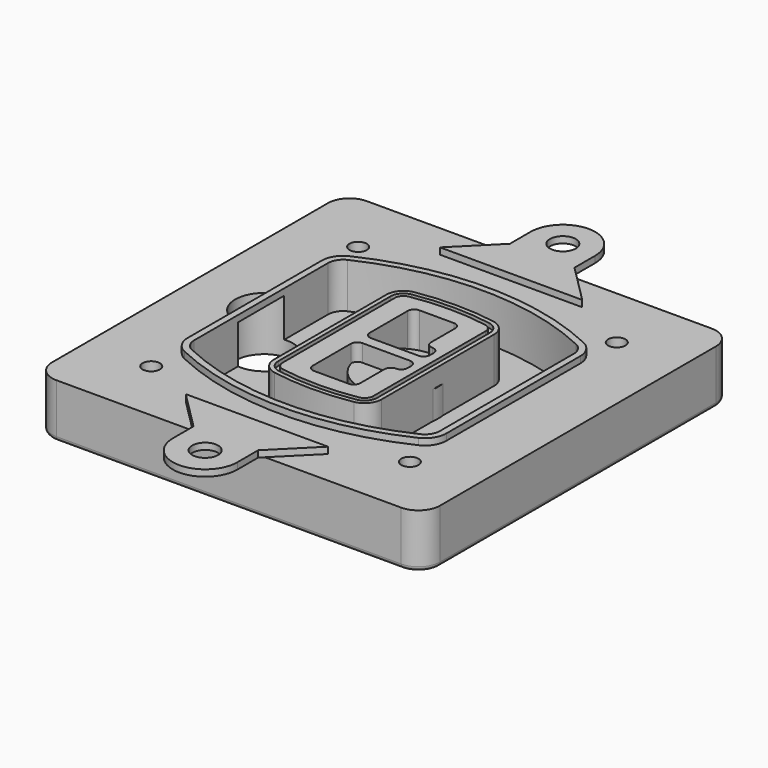
from build123d import *

# Parameters (mm, degrees)
F0_R      = 4
F1_DEPTH  = 25
F2_DEPTH  = 3
F3_DEPTH  = 18
F5_DEPTH  = 21
F6_DEPTH  = 2
F8_DEPTH  = 20
F9_DEPTH  = 16
F10_DEPTH = 25
F7_R      = 6
F7_R_2    = 4
F11_DEPTH = 6
F13_DEPTH = 9
F15_R     = 2
F16_R     = 6
F17_DEPTH = 3


# Not quite as in the source:
# - a feature of the source that left no trace in its solid (it failed there, or was rolled back) is left out
# - a feature names something its author has since deleted; it is built from what else it names


with BuildPart() as f1:
    # F0 (on Top) → F1 (new body)
    with BuildSketch(Plane.XY):
        with BuildLine():
            ThreePointArc((-90, -80), (-87.0710678119, -87.0710678119), (-80, -90))
            Line((-80, -90), (80, -90))
            ThreePointArc((80, -90), (87.0710678119, -87.0710678119), (90, -80))
            Line((90, -80), (90, 80))
            ThreePointArc((90, 80), (87.0710678119, 87.0710678119), (80, 90))
            Line((80, 90), (-80, 90))
            ThreePointArc((-80, 90), (-87.0710678119, 87.0710678119), (-90, 80))
            Line((-90, 80), (-90, -80))
        make_face()
        with Locations((-60, -60)):
            Circle(F0_R, mode=Mode.SUBTRACT)
        with Locations((60, -60)):
            Circle(F0_R, mode=Mode.SUBTRACT)
        with BuildLine():
            ThreePointArc((-64, 38.8308515907), (-61.8195654598, 46.3340424013), (-55.9574468085, 51.5000594398))
            ThreePointArc((-55.9574468085, 51.5000594398), (0, 64), (55.9574468085, 51.5000594398))
            ThreePointArc((55.9574468085, 51.5000594398), (61.8195654598, 46.3340424013), (64, 38.8308515907))
            Line((64, 38.8308515907), (64, -38.8308515907))
            ThreePointArc((64, -38.8308515907), (61.8195654598, -46.3340424013), (55.9574468085, -51.5000594398))
            ThreePointArc((55.9574468085, -51.5000594398), (0, -64), (-55.9574468085, -51.5000594398))
            ThreePointArc((-55.9574468085, -51.5000594398), (-61.8195654598, -46.3340424013), (-64, -38.8308515907))
            Line((-64, -38.8308515907), (-64, 38.8308515907))
        make_face(mode=Mode.SUBTRACT)
        with Locations((-60, 60)):
            Circle(F0_R, mode=Mode.SUBTRACT)
        with Locations((60, 60)):
            Circle(F0_R, mode=Mode.SUBTRACT)
        with BuildLine():
            ThreePointArc((55.9574468085, 51.5000594398), (0, 64), (-55.9574468085, 51.5000594398))
            ThreePointArc((-55.9574468085, 51.5000594398), (-61.8195654598, 46.3340424013), (-64, 38.8308515907))
            Line((-64, 38.8308515907), (-64, -38.8308515907))
            ThreePointArc((-64, -38.8308515907), (-61.8195654598, -46.3340424013), (-55.9574468085, -51.5000594398))
            ThreePointArc((-55.9574468085, -51.5000594398), (0, -64), (55.9574468085, -51.5000594398))
            ThreePointArc((55.9574468085, -51.5000594398), (61.8195654598, -46.3340424013), (64, -38.8308515907))
            Line((64, -38.8308515907), (64, 38.8308515907))
            ThreePointArc((64, 38.8308515907), (61.8195654598, 46.3340424013), (55.9574468085, 51.5000594398))
        make_face()
        with BuildLine():
            Line((-60, -38.8308515907), (-60, 38.8308515907))
            ThreePointArc((-60, 38.8308515907), (-58.442546757, 44.1902735983), (-54.2553191489, 47.8802857686))
            ThreePointArc((-54.2553191489, 47.8802857686), (0, 60), (54.2553191489, 47.8802857686))
            ThreePointArc((54.2553191489, 47.8802857686), (58.442546757, 44.1902735983), (60, 38.8308515907))
            Line((60, 38.8308515907), (60, -38.8308515907))
            ThreePointArc((60, -38.8308515907), (58.442546757, -44.1902735983), (54.2553191489, -47.8802857686))
            ThreePointArc((54.2553191489, -47.8802857686), (0, -60), (-54.2553191489, -47.8802857686))
            ThreePointArc((-54.2553191489, -47.8802857686), (-58.442546757, -44.1902735983), (-60, -38.8308515907))
        make_face(mode=Mode.SUBTRACT)
        with BuildLine():
            ThreePointArc((-54.2553191489, 47.8802857686), (-58.442546757, 44.1902735983), (-60, 38.8308515907))
            Line((-60, 38.8308515907), (-60, -38.8308515907))
            ThreePointArc((-60, -38.8308515907), (-58.442546757, -44.1902735983), (-54.2553191489, -47.8802857686))
            ThreePointArc((-54.2553191489, -47.8802857686), (0, -60), (54.2553191489, -47.8802857686))
            ThreePointArc((54.2553191489, -47.8802857686), (58.442546757, -44.1902735983), (60, -38.8308515907))
            Line((60, -38.8308515907), (60, 38.8308515907))
            ThreePointArc((60, 38.8308515907), (58.442546757, 44.1902735983), (54.2553191489, 47.8802857686))
            ThreePointArc((54.2553191489, 47.8802857686), (0, 60), (-54.2553191489, 47.8802857686))
        make_face()
        with BuildLine():
            ThreePointArc((52.9787234043, 45.1654555152), (55.9097827299, 42.582446996), (57, 38.8308515907))
            Line((57, 38.8308515907), (57, -38.8308515907))
            ThreePointArc((57, -38.8308515907), (55.9097827299, -42.582446996), (52.9787234043, -45.1654555152))
            ThreePointArc((52.9787234043, -45.1654555152), (0, -57), (-52.9787234043, -45.1654555152))
            ThreePointArc((-52.9787234043, -45.1654555152), (-55.9097827299, -42.582446996), (-57, -38.8308515907))
            Line((-57, -38.8308515907), (-57, 38.8308515907))
            ThreePointArc((-57, 38.8308515907), (-55.9097827299, 42.582446996), (-52.9787234043, 45.1654555152))
            ThreePointArc((-52.9787234043, 45.1654555152), (0, 57), (52.9787234043, 45.1654555152))
        make_face(mode=Mode.SUBTRACT)
        with BuildLine():
            Line((57, -38.8308515907), (57, 38.8308515907))
            ThreePointArc((57, 38.8308515907), (55.9097827299, 42.582446996), (52.9787234043, 45.1654555152))
            ThreePointArc((52.9787234043, 45.1654555152), (0, 57), (-52.9787234043, 45.1654555152))
            ThreePointArc((-52.9787234043, 45.1654555152), (-55.9097827299, 42.582446996), (-57, 38.8308515907))
            Line((-57, 38.8308515907), (-57, -38.8308515907))
            ThreePointArc((-57, -38.8308515907), (-55.9097827299, -42.582446996), (-52.9787234043, -45.1654555152))
            ThreePointArc((-52.9787234043, -45.1654555152), (0, -57), (52.9787234043, -45.1654555152))
            ThreePointArc((52.9787234043, -45.1654555152), (55.9097827299, -42.582446996), (57, -38.8308515907))
        make_face()
    extrude(amount=-F1_DEPTH)

    # F0 (on Top) → F2 (join)
    with BuildSketch(Plane.XY):
        with BuildLine():
            ThreePointArc((-54.2553191489, 47.8802857686), (-58.442546757, 44.1902735983), (-60, 38.8308515907))
            Line((-60, 38.8308515907), (-60, -38.8308515907))
            ThreePointArc((-60, -38.8308515907), (-58.442546757, -44.1902735983), (-54.2553191489, -47.8802857686))
            ThreePointArc((-54.2553191489, -47.8802857686), (0, -60), (54.2553191489, -47.8802857686))
            ThreePointArc((54.2553191489, -47.8802857686), (58.442546757, -44.1902735983), (60, -38.8308515907))
            Line((60, -38.8308515907), (60, 38.8308515907))
            ThreePointArc((60, 38.8308515907), (58.442546757, 44.1902735983), (54.2553191489, 47.8802857686))
            ThreePointArc((54.2553191489, 47.8802857686), (0, 60), (-54.2553191489, 47.8802857686))
        make_face()
        with BuildLine():
            ThreePointArc((52.9787234043, 45.1654555152), (55.9097827299, 42.582446996), (57, 38.8308515907))
            Line((57, 38.8308515907), (57, -38.8308515907))
            ThreePointArc((57, -38.8308515907), (55.9097827299, -42.582446996), (52.9787234043, -45.1654555152))
            ThreePointArc((52.9787234043, -45.1654555152), (0, -57), (-52.9787234043, -45.1654555152))
            ThreePointArc((-52.9787234043, -45.1654555152), (-55.9097827299, -42.582446996), (-57, -38.8308515907))
            Line((-57, -38.8308515907), (-57, 38.8308515907))
            ThreePointArc((-57, 38.8308515907), (-55.9097827299, 42.582446996), (-52.9787234043, 45.1654555152))
            ThreePointArc((-52.9787234043, 45.1654555152), (0, 57), (52.9787234043, 45.1654555152))
        make_face(mode=Mode.SUBTRACT)
    extrude(amount=F2_DEPTH)

    # F0 (on Top) → F3 (cut)
    with BuildSketch(Plane.XY):
        with BuildLine():
            Line((57, -38.8308515907), (57, 38.8308515907))
            ThreePointArc((57, 38.8308515907), (55.9097827299, 42.582446996), (52.9787234043, 45.1654555152))
            ThreePointArc((52.9787234043, 45.1654555152), (0, 57), (-52.9787234043, 45.1654555152))
            ThreePointArc((-52.9787234043, 45.1654555152), (-55.9097827299, 42.582446996), (-57, 38.8308515907))
            Line((-57, 38.8308515907), (-57, -38.8308515907))
            ThreePointArc((-57, -38.8308515907), (-55.9097827299, -42.582446996), (-52.9787234043, -45.1654555152))
            ThreePointArc((-52.9787234043, -45.1654555152), (0, -57), (52.9787234043, -45.1654555152))
            ThreePointArc((52.9787234043, -45.1654555152), (55.9097827299, -42.582446996), (57, -38.8308515907))
        make_face()
    extrude(amount=-F3_DEPTH, mode=Mode.SUBTRACT)

    # F4 (on face) → F5 (join, through all)
    with BuildSketch(Plane.XY.offset(3)):
        with BuildLine():
            ThreePointArc((-25, -32.5662280692), (-23.1122504785, -37.7276614059), (-18.3399014778, -40.4532214146))
            ThreePointArc((-18.3399014778, -40.4532214146), (0, -42), (18.3399014778, -40.4532214146))
            ThreePointArc((18.3399014778, -40.4532214146), (23.1122504785, -37.7276614059), (25, -32.5662280692))
            Line((25, -32.5662280692), (25, 32.5662280692))
            ThreePointArc((25, 32.5662280692), (23.1122504785, 37.7276614059), (18.3399014778, 40.4532214146))
            ThreePointArc((18.3399014778, 40.4532214146), (0, 42), (-18.3399014778, 40.4532214146))
            ThreePointArc((-18.3399014778, 40.4532214146), (-23.1122504785, 37.7276614059), (-25, 32.5662280692))
            Line((-25, 32.5662280692), (-25, -32.5662280692))
        make_face()
        with BuildLine():
            ThreePointArc((18.0049261084, 38.4814730782), (21.5841878588, 36.4373030717), (23, 32.5662280692))
            Line((23, 32.5662280692), (23, -32.5662280692))
            ThreePointArc((23, -32.5662280692), (21.5841878588, -36.4373030717), (18.0049261084, -38.4814730782))
            ThreePointArc((18.0049261084, -38.4814730782), (0, -40), (-18.0049261084, -38.4814730782))
            ThreePointArc((-18.0049261084, -38.4814730782), (-21.5841878588, -36.4373030717), (-23, -32.5662280692))
            Line((-23, -32.5662280692), (-23, 32.5662280692))
            ThreePointArc((-23, 32.5662280692), (-21.5841878588, 36.4373030717), (-18.0049261084, 38.4814730782))
            ThreePointArc((-18.0049261084, 38.4814730782), (0, 40), (18.0049261084, 38.4814730782))
        make_face(mode=Mode.SUBTRACT)
        with BuildLine():
            Line((23, -32.5662280692), (23, 32.5662280692))
            ThreePointArc((23, 32.5662280692), (21.5841878588, 36.4373030717), (18.0049261084, 38.4814730782))
            ThreePointArc((18.0049261084, 38.4814730782), (0, 40), (-18.0049261084, 38.4814730782))
            ThreePointArc((-18.0049261084, 38.4814730782), (-21.5841878588, 36.4373030717), (-23, 32.5662280692))
            Line((-23, 32.5662280692), (-23, -32.5662280692))
            ThreePointArc((-23, -32.5662280692), (-21.5841878588, -36.4373030717), (-18.0049261084, -38.4814730782))
            ThreePointArc((-18.0049261084, -38.4814730782), (0, -40), (18.0049261084, -38.4814730782))
            ThreePointArc((18.0049261084, -38.4814730782), (21.5841878588, -36.4373030717), (23, -32.5662280692))
        make_face()
        with BuildLine():
            ThreePointArc((17.6699507389, 36.5097247419), (20.0561252392, 35.1469447375), (21, 32.5662280692))
            Line((21, 32.5662280692), (21, -32.5662280692))
            ThreePointArc((21, -32.5662280692), (20.0561252392, -35.1469447375), (17.6699507389, -36.5097247419))
            ThreePointArc((17.6699507389, -36.5097247419), (0, -38), (-17.6699507389, -36.5097247419))
            ThreePointArc((-17.6699507389, -36.5097247419), (-20.0561252392, -35.1469447375), (-21, -32.5662280692))
            Line((-21, -32.5662280692), (-21, 32.5662280692))
            ThreePointArc((-21, 32.5662280692), (-20.0561252392, 35.1469447375), (-17.6699507389, 36.5097247419))
            ThreePointArc((-17.6699507389, 36.5097247419), (0, 38), (17.6699507389, 36.5097247419))
        make_face(mode=Mode.SUBTRACT)
        with BuildLine():
            Line((21, -32.5662280692), (21, 32.5662280692))
            ThreePointArc((21, 32.5662280692), (20.0561252392, 35.1469447375), (17.6699507389, 36.5097247419))
            ThreePointArc((17.6699507389, 36.5097247419), (0, 38), (-17.6699507389, 36.5097247419))
            ThreePointArc((-17.6699507389, 36.5097247419), (-20.0561252392, 35.1469447375), (-21, 32.5662280692))
            Line((-21, 32.5662280692), (-21, -32.5662280692))
            ThreePointArc((-21, -32.5662280692), (-20.0561252392, -35.1469447375), (-17.6699507389, -36.5097247419))
            ThreePointArc((-17.6699507389, -36.5097247419), (0, -38), (17.6699507389, -36.5097247419))
            ThreePointArc((17.6699507389, -36.5097247419), (20.0561252392, -35.1469447375), (21, -32.5662280692))
        make_face()
        with BuildLine():
            Line((-8, -2.5), (14, -2.5))
            ThreePointArc((14, -2.5), (16.1213203436, -3.3786796564), (17, -5.5))
            Line((17, -5.5), (17, -7.5))
            ThreePointArc((17, -7.5), (16.1213203436, -9.6213203436), (14, -10.5))
            ThreePointArc((14, -10.5), (11.8786796564, -11.3786796564), (11, -13.5))
            Line((11, -13.5), (11, -27.5))
            ThreePointArc((11, -27.5), (10.1213203436, -29.6213203436), (8, -30.5))
            Line((8, -30.5), (-8, -30.5))
            ThreePointArc((-8, -30.5), (-10.1213203436, -29.6213203436), (-11, -27.5))
            Line((-11, -27.5), (-11, -5.5))
            ThreePointArc((-11, -5.5), (-10.1213203436, -3.3786796564), (-8, -2.5))
        make_face(mode=Mode.SUBTRACT)
        with BuildLine():
            ThreePointArc((-8, 2.5), (-10.1213203436, 3.3786796564), (-11, 5.5))
            Line((-11, 5.5), (-11, 27.5))
            ThreePointArc((-11, 27.5), (-10.1213203436, 29.6213203436), (-8, 30.5))
            Line((-8, 30.5), (8, 30.5))
            ThreePointArc((8, 30.5), (10.1213203436, 29.6213203436), (11, 27.5))
            Line((11, 27.5), (11, 13.5))
            ThreePointArc((11, 13.5), (11.8786796564, 11.3786796564), (14, 10.5))
            ThreePointArc((14, 10.5), (16.1213203436, 9.6213203436), (17, 7.5))
            Line((17, 7.5), (17, 5.5))
            ThreePointArc((17, 5.5), (16.1213203436, 3.3786796564), (14, 2.5))
            Line((14, 2.5), (-8, 2.5))
        make_face(mode=Mode.SUBTRACT)
    extrude(amount=-F5_DEPTH)

    # F4 (on face) → F6 (cut)
    with BuildSketch(Plane.XY.offset(3)):
        with BuildLine():
            Line((23, -32.5662280692), (23, 32.5662280692))
            ThreePointArc((23, 32.5662280692), (21.5841878588, 36.4373030717), (18.0049261084, 38.4814730782))
            ThreePointArc((18.0049261084, 38.4814730782), (0, 40), (-18.0049261084, 38.4814730782))
            ThreePointArc((-18.0049261084, 38.4814730782), (-21.5841878588, 36.4373030717), (-23, 32.5662280692))
            Line((-23, 32.5662280692), (-23, -32.5662280692))
            ThreePointArc((-23, -32.5662280692), (-21.5841878588, -36.4373030717), (-18.0049261084, -38.4814730782))
            ThreePointArc((-18.0049261084, -38.4814730782), (0, -40), (18.0049261084, -38.4814730782))
            ThreePointArc((18.0049261084, -38.4814730782), (21.5841878588, -36.4373030717), (23, -32.5662280692))
        make_face()
        with BuildLine():
            ThreePointArc((17.6699507389, 36.5097247419), (20.0561252392, 35.1469447375), (21, 32.5662280692))
            Line((21, 32.5662280692), (21, -32.5662280692))
            ThreePointArc((21, -32.5662280692), (20.0561252392, -35.1469447375), (17.6699507389, -36.5097247419))
            ThreePointArc((17.6699507389, -36.5097247419), (0, -38), (-17.6699507389, -36.5097247419))
            ThreePointArc((-17.6699507389, -36.5097247419), (-20.0561252392, -35.1469447375), (-21, -32.5662280692))
            Line((-21, -32.5662280692), (-21, 32.5662280692))
            ThreePointArc((-21, 32.5662280692), (-20.0561252392, 35.1469447375), (-17.6699507389, 36.5097247419))
            ThreePointArc((-17.6699507389, 36.5097247419), (0, 38), (17.6699507389, 36.5097247419))
        make_face(mode=Mode.SUBTRACT)
    extrude(amount=-F6_DEPTH, mode=Mode.SUBTRACT)

    # F7 (on face) → F8 (join)
    with BuildSketch(Plane(origin=(0, 0, -25), x_dir=(1, 0, 0), z_dir=(0, 0, -1))):
        with BuildLine():
            ThreePointArc((-6.71157564, 0), (6.7567035675, 13.4682792075), (20.224982775, 0))
            Line((20.224982775, 0), (25.224982775, 0))
            ThreePointArc((25.224982775, 0), (6.7567035675, 18.4682792075), (-11.71157564, 0))
            Line((-11.71157564, 0), (-6.71157564, 0))
        make_face()
        with BuildLine():
            Line((-6.71157564, 0), (20.224982775, 0))
            ThreePointArc((20.224982775, 0), (6.7567035675, 13.4682792075), (-6.71157564, 0))
        make_face()
        with BuildLine():
            ThreePointArc((-6.71157564, 0), (6.7567035675, -13.4682792075), (20.224982775, 0))
            Line((20.224982775, 0), (-6.71157564, 0))
        make_face()
        with BuildLine():
            Line((25.224982775, 0), (20.224982775, 0))
            ThreePointArc((20.224982775, 0), (6.7567035675, -13.4682792075), (-6.71157564, 0))
            Line((-6.71157564, 0), (-11.71157564, 0))
            ThreePointArc((-11.71157564, 0), (6.7567035675, -18.4682792075), (25.224982775, 0))
        make_face()
    extrude(amount=-F8_DEPTH)

    # F7 (on face) → F9 (cut)
    with BuildSketch(Plane(origin=(0, 0, -25), x_dir=(1, 0, 0), z_dir=(0, 0, -1))):
        with BuildLine():
            Line((-6.71157564, 0), (20.224982775, 0))
            ThreePointArc((20.224982775, 0), (6.7567035675, 13.4682792075), (-6.71157564, 0))
        make_face()
        with BuildLine():
            ThreePointArc((-6.71157564, 0), (6.7567035675, -13.4682792075), (20.224982775, 0))
            Line((20.224982775, 0), (-6.71157564, 0))
        make_face()
    extrude(amount=-F9_DEPTH, mode=Mode.SUBTRACT)

    # F7 (on face) → F10 (cut)
    with BuildSketch(Plane(origin=(0, 0, -25), x_dir=(1, 0, 0), z_dir=(0, 0, -1))):
        with BuildLine():
            Line((-69.0318229325, 0), (-42.0952645175, 0))
            ThreePointArc((-42.0952645175, 0), (-55.563543725, 13.4682792075), (-69.0318229325, 0))
        make_face()
        with BuildLine():
            ThreePointArc((-69.0318229325, 0), (-55.563543725, -13.4682792075), (-42.0952645175, 0))
            Line((-42.0952645175, 0), (-69.0318229325, 0))
        make_face()
    extrude(amount=-F10_DEPTH, mode=Mode.SUBTRACT)

    # F7 (on face) → F11 (cut)
    with BuildSketch(Plane(origin=(0, 0, -25), x_dir=(1, 0, 0), z_dir=(0, 0, -1))):
        with Locations((60, -60)):
            Circle(F7_R)
        with Locations((60, -60)):
            Circle(F7_R_2, mode=Mode.SUBTRACT)
        with Locations((-60, -60)):
            Circle(F7_R)
        with Locations((-60, -60)):
            Circle(F7_R_2, mode=Mode.SUBTRACT)
        with Locations((-60, 60)):
            Circle(F7_R)
        with Locations((-60, 60)):
            Circle(F7_R_2, mode=Mode.SUBTRACT)
        with Locations((60, 60)):
            Circle(F7_R)
        with Locations((60, 60)):
            Circle(F7_R_2, mode=Mode.SUBTRACT)
    extrude(amount=-F11_DEPTH, mode=Mode.SUBTRACT)

    # F12 (on face) → F13 (cut, through all)
    with BuildSketch(Plane(origin=(0, 0, -9), x_dir=(1, 0, 0), z_dir=(0, 0, -1))):
        with BuildLine():
            ThreePointArc((20.224982775, 0), (20.1663399806, 1.2554664788), (19.9909222755, 2.5))
            Line((19.9909222755, 2.5), (14, 2.5))
            ThreePointArc((14, 2.5), (16.1213203436, 3.3786796564), (17, 5.5))
            Line((17, 5.5), (17, 7.5))
            ThreePointArc((17, 7.5), (16.1213203436, 9.6213203436), (14, 10.5))
            ThreePointArc((14, 10.5), (12.1627255951, 11.1284134507), (11.0951631559, 12.750384826))
            ThreePointArc((11.0951631559, 12.750384826), (11.0476113807, 12.7664660322), (11, 12.7823698976))
            Line((11, 12.7823698976), (11, -12.7823698976))
            ThreePointArc((11, -12.7823698976), (11.0476113807, -12.7664660322), (11.0951631559, -12.750384826))
            ThreePointArc((11.0951631559, -12.750384826), (12.1627255951, -11.1284134507), (14, -10.5))
            ThreePointArc((14, -10.5), (16.1213203436, -9.6213203436), (17, -7.5))
            Line((17, -7.5), (17, -5.5))
            ThreePointArc((17, -5.5), (16.1213203436, -3.3786796564), (14, -2.5))
            Line((14, -2.5), (19.9909222755, -2.5))
            ThreePointArc((19.9909222755, -2.5), (20.1663399806, -1.2554664788), (20.224982775, 0))
        make_face()
    extrude(amount=F13_DEPTH, mode=Mode.SUBTRACT)

    # F15
    f15_edges = [f1.edges().sort_by_distance(p)[0] for p in [
        (0, -90, -25),
        (-87.071068, -87.071068, -25),
        (-90, 0, -25),
        (-87.071068, 87.071068, -25),
        (87.071068, -87.071068, -25),
        (0, 90, -25),
        (90, 0, -25),
        (87.071068, 87.071068, -25),
    ]]
    fillet(f15_edges, radius=F15_R)


with BuildPart() as f17:
    # F16 (on Top) → F17 (new body, through all)
    with BuildSketch(Plane.XY):
        with BuildLine():
            Line((-15, 91.7296429276), (-33, 73.7296429276))
            Line((-33, 73.7296429276), (33, 73.7296429276))
            Line((33, 73.7296429276), (15, 91.7296429276))
            Line((15, 91.7296429276), (15, 103.7296429276))
            ThreePointArc((15, 103.7296429276), (0, 118.7296429276), (-15, 103.7296429276))
            Line((-15, 103.7296429276), (-15, 91.7296429276))
        make_face()
        with Locations((0, 103.7296429276)):
            Circle(F16_R, mode=Mode.SUBTRACT)
    extrude(amount=F17_DEPTH)


with BuildPart() as f17b:
    # F16 (on Top) → F17, piece 2 (new body, through all)
    with BuildSketch(Plane.XY):
        with BuildLine():
            ThreePointArc((-15, -103.7296429276), (0, -118.7296429276), (15, -103.7296429276))
            Line((15, -103.7296429276), (15, -91.7296429276))
            Line((15, -91.7296429276), (33, -73.7296429276))
            Line((33, -73.7296429276), (-33, -73.7296429276))
            Line((-33, -73.7296429276), (-15, -91.7296429276))
            Line((-15, -91.7296429276), (-15, -103.7296429276))
        make_face()
        with Locations((0, -103.7296429276)):
            Circle(F16_R, mode=Mode.SUBTRACT)
    extrude(amount=F17_DEPTH)


solid = Compound([f1.part, f17.part, f17b.part])
